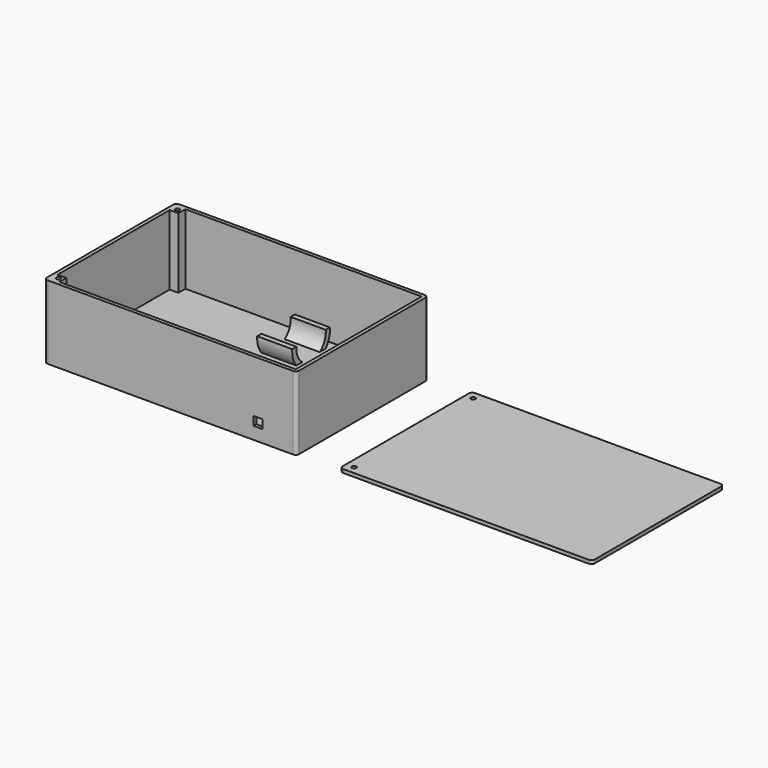
from build123d import *

# Parameters (mm, degrees)
F0_R      = 1.25
F1_DEPTH  = 2
F0_W      = 5
F0_H      = 5
F2_DEPTH  = 42
F4_DEPTH  = 20
F6_D      = 2.5
F6_DEPTH  = 100
F6_TIP    = 0.7510757738
F5_R      = 1.25
F7_DEPTH  = 2
F9_W      = 5
F9_H      = 5
F10_DEPTH = 254


# Not quite as in the source:
# - ends of sketch curves that miss each other by under 0.0002 mm in the source are joined


with BuildPart() as f1:
    # F0 (on Top) → F1 (new body)
    with BuildSketch(Plane.XY):
        Polygon((70, -45), (70, 45), (-65, 45), (-65, 40), (-70, 40), (-70, -40), (-65, -40), (-65, -45), align=None)
        with Locations((-6.5, -40)):
            Circle(F0_R, mode=Mode.SUBTRACT)
        with Locations((65, -35)):
            Circle(F0_R, mode=Mode.SUBTRACT)
        with Locations((65, -6.5)):
            Circle(F0_R, mode=Mode.SUBTRACT)
        with Locations((-6.5, 9)):
            Circle(F0_R, mode=Mode.SUBTRACT)
    extrude(amount=F1_DEPTH)

    # F0 (on Top) → F2 (join)
    with BuildSketch(Plane.XY):
        with BuildLine():
            ThreePointArc((72, 45), (71.4142135624, 46.4142135624), (70, 47))
            Line((70, 47), (-70, 47))
            ThreePointArc((-70, 47), (-71.4142135624, 46.4142135624), (-72, 45))
            Line((-72, 45), (-72, -45))
            ThreePointArc((-72, -45), (-71.4142135624, -46.4142135624), (-70, -47))
            Line((-70, -47), (70, -47))
            ThreePointArc((70, -47), (71.4142135624, -46.4142135624), (72, -45))
            Line((72, -45), (72, 45))
        make_face()
        Polygon((-65, 45), (70, 45), (70, -45), (-65, -45), (-70, -45), (-70, -40), (-70, 40), (-70, 45), align=None, mode=Mode.SUBTRACT)
        with Locations((-67.5, 42.5)):
            Rectangle(F0_W, F0_H)
        with Locations((-67.5, -42.5)):
            Rectangle(F0_W, F0_H)
    extrude(amount=F2_DEPTH)

    # F3 (on Right) → F4 (join)
    with BuildSketch(Plane.YZ):
        with BuildLine():
            Line((19.9825780445, 0), (20.0136909165, 0))
            Line((20.0136909165, 0), (28.5, 0))
            ThreePointArc((28.5, 0), (20.7214244856, 3.411512363), (18.0097533873, 11.4608090371))
            Line((18.0097533873, 11.4608090371), (15, 11.4608090371))
            ThreePointArc((15, 11.4608090371), (16.0856243868, 5.1192928834), (19.9825780445, 0))
        make_face()
        with BuildLine():
            ThreePointArc((38.9280208686, 11.4608090371), (36.2373225983, 3.4344937669), (28.4999998635, 4.60827e-05))
            Line((28.4999998635, 4.60827e-05), (36.9551962114, 0))
            ThreePointArc((36.9551962114, 0), (40.8521498691, 5.1192928834), (41.9377742559, 11.4608090371))
            Line((41.9377742559, 11.4608090371), (38.9280208686, 11.4608090371))
        make_face()
    extrude(amount=F4_DEPTH)

    # F6
    with Locations(Plane(origin=(0, 0, 0), x_dir=(1, 0, 0), z_dir=(0, 0, -1))):
        with Locations((-67.5, -42.5), (-67.5, 42.5)):
            Hole(F6_D / 2, depth=F6_DEPTH)
            with Locations((0, 0, -(F6_DEPTH + F6_TIP / 2))):  # 118° drill point
                Cone(0, F6_D / 2, F6_TIP, mode=Mode.SUBTRACT)

    # F9 (on face) → F10 (cut)
    with BuildSketch(Plane.XZ.offset(47)):
        with Locations((50, 9.5896283165)):
            Rectangle(F9_W, F9_H)
    extrude(amount=-F10_DEPTH, mode=Mode.SUBTRACT)


with BuildPart() as f7:
    # F5 (on face) → F7 (new body)
    with BuildSketch(Plane.XY.offset(42)):
        with BuildLine():
            ThreePointArc((240.829995513, 45.0000016093), (240.2442090753, 46.4142151717), (238.829995513, 47.0000016093))
            Line((238.829995513, 47.0000016093), (98.829995513, 47.0000016093))
            ThreePointArc((98.829995513, 47.0000016093), (97.4157819506, 46.4142151717), (96.829995513, 45.0000016093))
            Line((96.829995513, 45.0000016093), (96.829995513, -44.9999983907))
            ThreePointArc((96.829995513, -44.9999983907), (97.4157819506, -46.414211953), (98.829995513, -46.9999983907))
            Line((98.829995513, -46.9999983907), (238.829995513, -46.9999983907))
            ThreePointArc((238.829995513, -46.9999983907), (240.2442090753, -46.414211953), (240.829995513, -44.9999983907))
            Line((240.829995513, -44.9999983907), (240.829995513, 45.0000016093))
        make_face()
        with Locations((101.325795513, -42.5041983907)):
            Circle(F5_R, mode=Mode.SUBTRACT)
        with Locations((101.3298566341, 42.500115931)):
            Circle(F5_R, mode=Mode.SUBTRACT)
    extrude(amount=F7_DEPTH)


with BuildPart() as f7_1:
    # F8: moved
    add(f7.part.moved(Location((0, 0, -42))))


solid = Compound([f1.part, f7_1.part])
